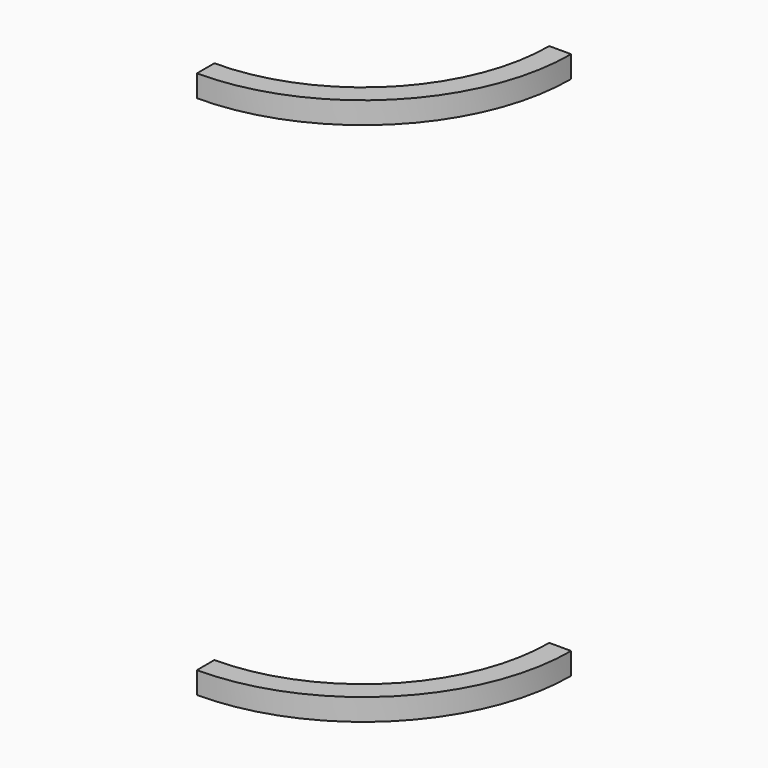
from build123d import *

# Parameters (mm, degrees)
F3_ANGLE = 90


# Not quite as in the source:
# - a feature names something its author has since deleted; it is built from what else it names
# - the program builds the solid bodies; features that only make, move or delete a surface that nothing else refers to are left out


with BuildPart() as f3:
    # F2 (on Front) → F3 (revolve)
    with BuildSketch(Plane.XZ):
        Polygon((40.834482817, 48.9924472272), (36.834482817, 48.9924472272), (36.834482817, 46.9924472272), (38.834482817, 46.9924472272), (38.834482817, 44.9924472272), (40.834482817, 44.9924472272), (40.834482817, 46.9924472272), align=None)
    revolve(axis=Axis((2.834482817, 0, 46.6319954246), (0, 0, -1)), revolution_arc=F3_ANGLE)


with BuildPart() as f4_1:
    # F4: copy of F3
    add(f3.part)


with BuildPart() as f3_1:
    # F5: moved
    add(f3.part.moved(Location((0, 0, -100))))


with BuildPart() as f3_2:
    # F6: moved
    add(f3_1.part.moved(Location((0, 30, 4))))


with BuildPart() as f3_3:
    # F7: moved
    add(f3_2.part.moved(Location((0, -30, 0))))


solid = Compound([f4_1.part, f3_3.part])
